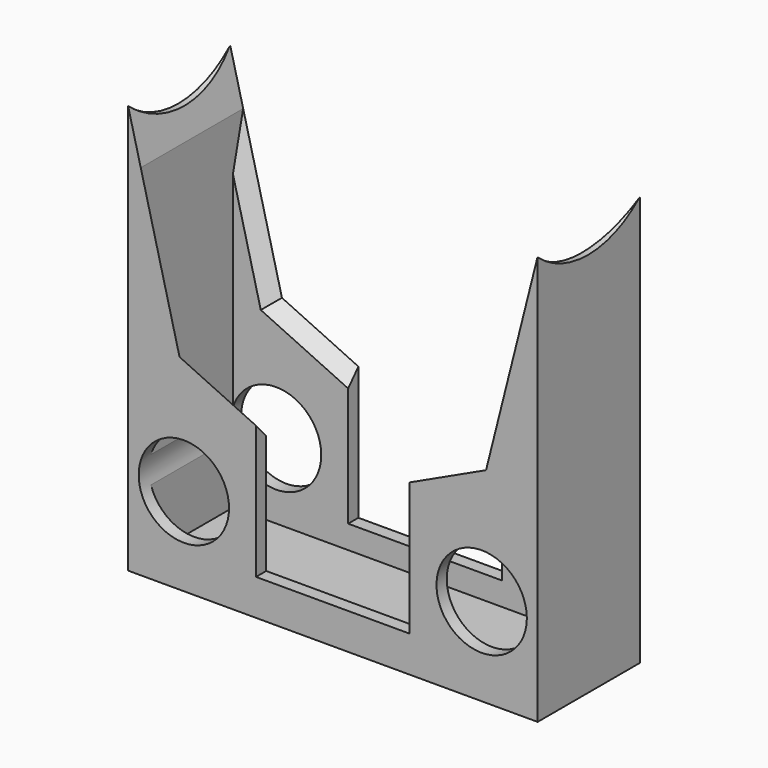
from build123d import *

# Parameters (mm, degrees)
F1_DEPTH      = 25.4
F2_T          = -2.54
F3_R          = 8.9609270722
F4_DEPTH      = 105.41
F5_SIZE       = 2.53999
F6_R          = 19.1294081244
F7_DEPTH      = 254
F7_DEPTH_BACK = 170.942


# Not quite as in the source:
# - a fillet or chamfer is up to 0.001 mm smaller than in the source, because OpenCascade refuses the exact size


with BuildPart() as f1:
    # F0 (on Front) → F1 (new body)
    with BuildSketch(Plane.XZ):
        Polygon((40.64, -40.64), (40.64, 0), (30.4068718106, 0), (15.24, -7.0667252876), (15.24, -33.4807746112), (-15.24, -33.4807746112), (-15.24, -7.0667252876), (-30.4068718106, 0), (-40.64, 0), (-40.64, -40.64), align=None)
        Polygon((-30.4068718106, 0), (-40.64, 40.64), (-40.64, 0), align=None)
        Polygon((40.64, 0), (40.64, 40.64), (30.4068718106, 0), align=None)
    extrude(amount=F1_DEPTH)

    # F2
    f2_openings = [f1.faces().sort_by_distance(p)[0] for p in [
        (35.523436, -12.7, 20.32),
        (22.823436, -12.7, -3.533363),
        (15.24, -12.7, -20.27375),
        (0, -12.7, -33.480775),
        (-35.523436, -12.7, 20.32),
        (-22.823436, -12.7, -3.533363),
        (-15.24, -12.7, -20.27375),
    ]]
    offset(amount=F2_T, openings=f2_openings)

    # F3 (on Front) → F4 (cut)
    with BuildSketch(Plane.XZ):
        with Locations((-29.5430510807, -23.22207205)):
            Circle(F3_R)
        with Locations((29.538249597, -23.22207205)):
            Circle(F3_R)
    extrude(amount=F4_DEPTH, mode=Mode.SUBTRACT)

    # F5 (size 2.54 in the source; OpenCascade refuses exactly that, so slightly less here)
    f5_edges = [f1.edges().sort_by_distance(p)[0] for p in [
        (-34.253436, -22.86, 15.276303),
        (-22.823436, -22.86, -3.533363),
        (-34.253436, -2.54, 15.276303),
        (-22.823436, -2.54, -3.533363),
        (22.823436, -2.54, -3.533363),
        (34.253436, -2.54, 15.276303),
        (34.253436, -22.86, 15.276303),
        (22.823436, -22.86, -3.533363),
    ]]
    chamfer(f5_edges, length=F5_SIZE)

    # F6 (on Right) → F7 (cut, two sides)
    with BuildSketch(Plane.YZ) as f7_sk:
        with Locations((-12.8998877481, 54.9755766988)):
            Circle(F6_R)
    extrude(amount=-F7_DEPTH, mode=Mode.SUBTRACT)
    extrude(f7_sk.sketch, amount=F7_DEPTH_BACK, mode=Mode.SUBTRACT)


solid = f1.part
